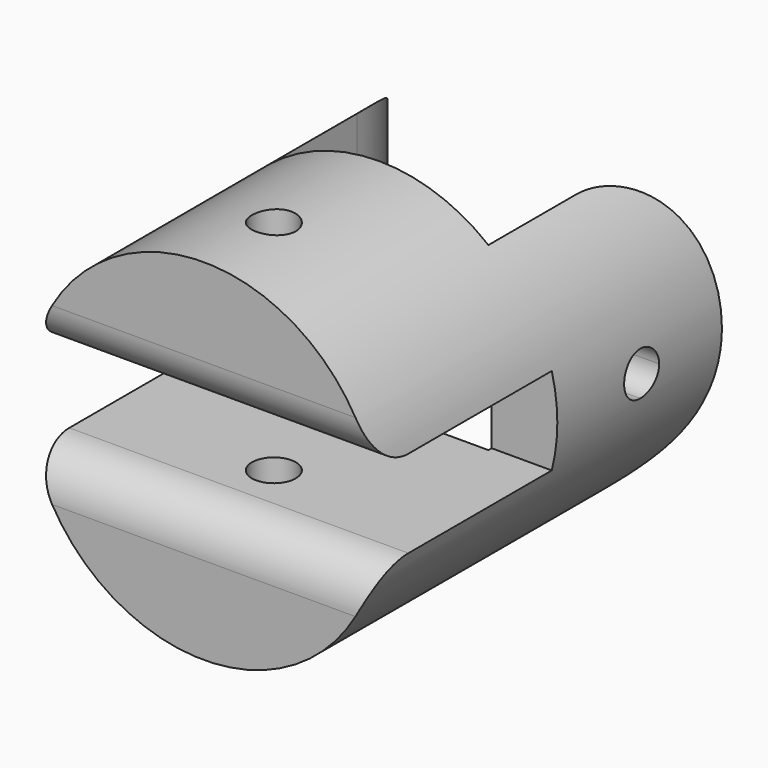
from build123d import *

# Parameters (mm, degrees)
F0_R        = 8
F1_DEPTH    = 20
F2_W        = 10
F2_H        = 20.4895668926
F3_DEPTH    = 10
F4_W        = 20
F4_H        = 4
F5_DEPTH    = 50
F6_T1_DEPTH = 37.4899959968
F7_R        = 2
F9_DEPTH    = 50
F10_R       = 1
F11_DEPTH   = 25


# Not quite as in the source:
# - a fillet or chamfer that OpenCascade refuses, or shapes differently, is made with other operations: its cross-section is extruded or revolved along the edge and cut away or added


with BuildPart() as f1:
    # F0 (on Front) → F1 (new body)
    with BuildSketch(Plane.XZ):
        Circle(F0_R)
    extrude(amount=F1_DEPTH)

    # F2 (on Front) → F3 (cut)
    with BuildSketch(Plane.XZ):
        Rectangle(F2_W, F2_H)
    extrude(amount=F3_DEPTH, mode=Mode.SUBTRACT)

    # F4 (on Right) → F5 (cut, symmetric)
    with BuildSketch(Plane.YZ):
        with Locations((-19.8148275974, 0)):
            Rectangle(F4_W, F4_H)
    extrude(amount=F5_DEPTH, both=True, mode=Mode.SUBTRACT)

    # F6: fillet of radius 5 on 2 edges, made by hand

    # F6_s2 → F6_t1 (cut)
    with BuildSketch(Plane.XY.offset(-18.7449979984)):
        with BuildLine():
            ThreePointArc((10, 0), (6.4644660941, -1.4644660941), (5, -5))
            Line((5, -5), (5, 0))
            Line((5, 0), (10, 0))
        make_face()
        with BuildLine():
            ThreePointArc((-5, -5), (-6.4644660941, -1.4644660941), (-10, 0))
            Line((-10, 0), (-5, 0))
            Line((-5, 0), (-5, -5))
        make_face()
    extrude(amount=F6_T1_DEPTH, mode=Mode.SUBTRACT)

    # F7
    f7_edges = [f1.edges().sort_by_distance(p)[0] for p in [
        (0, -20, -2),
        (0, -20, 2),
    ]]
    fillet(f7_edges, radius=F7_R)

    # F8 (on face) → F9 (cut, symmetric)
    with BuildSketch(Plane.YZ.offset(-5)):
        with BuildLine():
            Line((-5, -1), (-5, 1))
            ThreePointArc((-5, 1), (-6, 0), (-5, -1))
        make_face()
        with BuildLine():
            ThreePointArc((-5, -1), (-4.2928932188, -0.7071067812), (-4, 0))
            ThreePointArc((-4, 0), (-4.2928932188, 0.7071067812), (-5, 1))
            Line((-5, 1), (-5, -1))
        make_face()
    extrude(amount=F9_DEPTH, both=True, mode=Mode.SUBTRACT)

    # F10 (on Top) → F11 (cut, symmetric)
    with BuildSketch(Plane.XY):
        with Locations((0, -16)):
            Circle(F10_R)
    extrude(amount=F11_DEPTH, both=True, mode=Mode.SUBTRACT)


solid = f1.part
